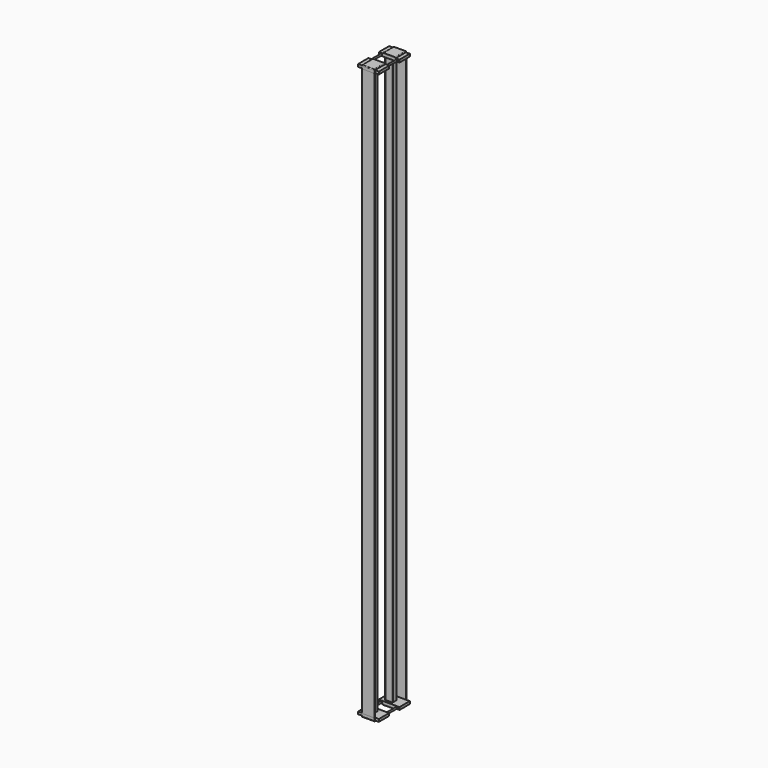
from build123d import *

# Parameters (mm, degrees)
F1_W     = 80
F1_H     = 10
F2_DEPTH = 50
F4_R     = 3
F5_DEPTH = 80
F7_DEPTH = 1100
F9_DEPTH = 25
F11_R    = 2.99999
F11_2_R  = 2.99999
F11_3_R  = 2.99999
F11_4_R  = 2.99999


# Not quite as in the source:
# - a fillet or chamfer is up to 0.001 mm smaller than in the source, because OpenCascade refuses the exact size
# - a feature names something its author has since deleted; it is built from what else it names


with BuildPart() as f2:
    # F1 (on offset) → F2 (new body)
    with BuildSketch(Plane.XZ.offset(25)):
        with Locations((0, 1105)):
            Rectangle(F1_W, F1_H)
    extrude(amount=F2_DEPTH)


with BuildPart() as f2b:
    # F1 (on offset) → F2, piece 2 (new body)
    with BuildSketch(Plane.XZ.offset(25)):
        with Locations((0, -1105)):
            Rectangle(F1_W, F1_H)
    extrude(amount=F2_DEPTH)


with BuildPart() as f5:
    # F4 (on face) → F5 (new body)
    with BuildSketch(Plane(origin=(0, -25, 0), x_dir=(-1, 0, 0), z_dir=(0, 1, 0))):
        with Locations((-30, 1105)):
            Circle(F4_R)
    extrude(amount=F5_DEPTH)


with BuildPart() as f5b:
    # F4 (on face) → F5, piece 2 (new body)
    with BuildSketch(Plane(origin=(0, -25, 0), x_dir=(-1, 0, 0), z_dir=(0, 1, 0))):
        with Locations((30, 1105)):
            Circle(F4_R)
    extrude(amount=F5_DEPTH)


with BuildPart() as f5c:
    # F4 (on face) → F5, piece 3 (new body)
    with BuildSketch(Plane(origin=(0, -25, 0), x_dir=(-1, 0, 0), z_dir=(0, 1, 0))):
        with Locations((-30, -1105)):
            Circle(F4_R)
    extrude(amount=F5_DEPTH)


with BuildPart() as f5d:
    # F4 (on face) → F5, piece 4 (new body)
    with BuildSketch(Plane(origin=(0, -25, 0), x_dir=(-1, 0, 0), z_dir=(0, 1, 0))):
        with Locations((30, -1105)):
            Circle(F4_R)
    extrude(amount=F5_DEPTH)


with BuildPart() as f7:
    # F6 (on Top) → F7 (new body, symmetric)
    with BuildSketch(Plane.XY):
        with BuildLine():
            Line((-25, -38), (-25, -75))
            ThreePointArc((-25, -75), (-24.1213203436, -77.1213203436), (-22, -78))
            Line((-22, -78), (25, -78))
            Line((25, -78), (25, -75))
            Line((25, -75), (-22, -75))
            Line((-22, -75), (-22, -38))
            Line((-22, -38), (2, -38))
            Line((2, -38), (2, -55))
            Line((2, -55), (5, -55))
            Line((5, -55), (5, -38))
            ThreePointArc((5, -38), (4.1213203436, -35.8786796564), (2, -35))
            Line((2, -35), (-22, -35))
            ThreePointArc((-22, -35), (-24.1213203436, -35.8786796564), (-25, -38))
        make_face()
    extrude(amount=F7_DEPTH, both=True)


with BuildPart() as f9:
    # F8 (on Right) → F9 (new body, symmetric)
    with BuildSketch(Plane.YZ):
        with BuildLine():
            Line((-75, -1110), (-75, -1100))
            Line((-75, -1100), (-78, -1100))
            Line((-78, -1100), (-78, -1110))
            ThreePointArc((-78, -1110), (-77.1213203436, -1112.1213203436), (-75, -1113))
            Line((-75, -1113), (-25, -1113))
            Line((-25, -1113), (-25, -1110))
            Line((-25, -1110), (-75, -1110))
        make_face()
    extrude(amount=F9_DEPTH, both=True)


with BuildPart() as f9b:
    # F8 (on Right) → F9, piece 2 (new body, symmetric)
    with BuildSketch(Plane.YZ):
        with BuildLine():
            ThreePointArc((-75, 1113), (-77.1213203436, 1112.1213203436), (-78, 1110))
            Line((-78, 1110), (-78, 1100))
            Line((-78, 1100), (-75, 1100))
            Line((-75, 1100), (-75, 1110))
            Line((-75, 1110), (-25, 1110))
            Line((-25, 1110), (-25, 1113))
            Line((-25, 1113), (-75, 1113))
        make_face()
    extrude(amount=F9_DEPTH, both=True)


with BuildPart() as f10_1:
    # F10: instance of F2
    add(f2.part.mirror(Plane.XZ))


with BuildPart() as f10_2:
    # F10: instance of F2b
    add(f2b.part.mirror(Plane.XZ))


with BuildPart() as f10_3:
    # F10: instance of F7
    add(f7.part.mirror(Plane.XZ))


with BuildPart() as f10_4:
    # F10: instance of F9b
    add(f9b.part.mirror(Plane.XZ))

    # F11#3 (radius 3 in the source; OpenCascade refuses exactly that, so slightly less here)
    f11_3_edges = [f10_4.edges().sort_by_distance(p)[0] for p in [
        (-25, 78, 1105),
        (25, 78, 1105),
        (-25, 77.12132, 1112.12132),
        (25, 77.12132, 1112.12132),
        (-25, 50, 1113),
        (25, 50, 1113),
    ]]
    fillet(f11_3_edges, radius=F11_3_R)


with BuildPart() as f10_5:
    # F10: instance of F9
    add(f9.part.mirror(Plane.XZ))

    # F11#4 (radius 3 in the source; OpenCascade refuses exactly that, so slightly less here)
    f11_4_edges = [f10_5.edges().sort_by_distance(p)[0] for p in [
        (-25, 50, -1113),
        (-25, 77.12132, -1112.12132),
        (-25, 78, -1105),
    ]]
    fillet(f11_4_edges, radius=F11_4_R)


with BuildPart() as f9_1:
    add(f9.part)

    # F11 (radius 3 in the source; OpenCascade refuses exactly that, so slightly less here)
    f11_edges = [f9_1.edges().sort_by_distance(p)[0] for p in [
        (-25, -78, -1105),
        (-25, -50, -1113),
        (-25, -77.12132, -1112.12132),
    ]]
    fillet(f11_edges, radius=F11_R)


with BuildPart() as f9b_1:
    add(f9b.part)

    # F11#2 (radius 3 in the source; OpenCascade refuses exactly that, so slightly less here)
    f11_2_edges = [f9b_1.edges().sort_by_distance(p)[0] for p in [
        (25, -50, 1113),
        (-25, -50, 1113),
        (-25, -78, 1105),
        (25, -78, 1105),
        (-25, -77.12132, 1112.12132),
        (25, -77.12132, 1112.12132),
    ]]
    fillet(f11_2_edges, radius=F11_2_R)


solid = Compound([f2.part, f2b.part, f5.part, f5b.part, f5c.part, f5d.part, f7.part, f10_1.part, f10_2.part, f10_3.part, f10_4.part, f10_5.part, f9_1.part, f9b_1.part])
